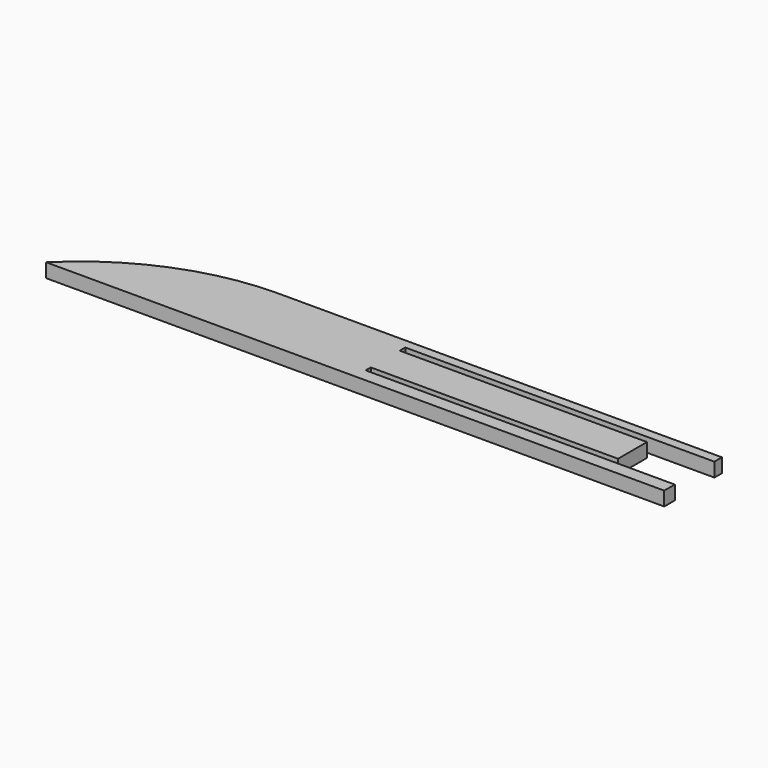
from build123d import *

# Parameters (mm, degrees)
F1_DEPTH    = 6
F2_DEPTH    = 0.8
F3_T1_DEPTH = 431.7925725323
F4_DEPTH    = 30


# Not quite as in the source:
# - a fillet or chamfer that OpenCascade refuses, or shapes differently, is made with other operations: its cross-section is extruded or revolved along the edge and cut away or added


with BuildPart() as f1:
    # F0 (on Top) → F1 (new body)
    with BuildSketch(Plane.XY):
        Polygon((150, 17.5), (-150, 17.5), (-150, -17.5), (150, -17.5), (150, -11.1123658717), (0, -11.1123658717), (0, -8.0123320222), (150, -8.0123320222), (150, 9.5545258373), (0, 9.5545258373), (0, 12.9128964618), (150, 12.9128964618), align=None)
    extrude(amount=F1_DEPTH)

    # F2 (add): faces of the model
    f2_faces = [f1.faces().sort_by_distance(p)[0] for p in [
        (-7.6230433236, -0.1272136786, 0),
        (-7.6230433236, -0.1272136786, 6),
    ]]
    extrude(f2_faces, amount=F2_DEPTH, dir=(0, 0, -1))

    # F3: fillet of radius 120.7106781187 on 1 edges, made by hand

    # F3_s2 → F3_t1 (cut)
    with BuildSketch(Plane.XY.offset(-213.2962862662)):
        with BuildLine():
            ThreePointArc((-65.0014854935, 17.5), (-110.9627394699, 8.4075593911), (-150, -17.5))
            Line((-150, -17.5), (-150, 17.5))
            Line((-150, 17.5), (-65.0014854935, 17.5))
        make_face()
    extrude(amount=F3_T1_DEPTH, mode=Mode.SUBTRACT)

    # F4 (cut): a face of the model
    f4_faces = [f1.faces().sort_by_distance(p)[0] for p in [
        (150, 0.7710969076, 2.6),
    ]]
    extrude(f4_faces, amount=-F4_DEPTH, mode=Mode.SUBTRACT)


solid = f1.part
